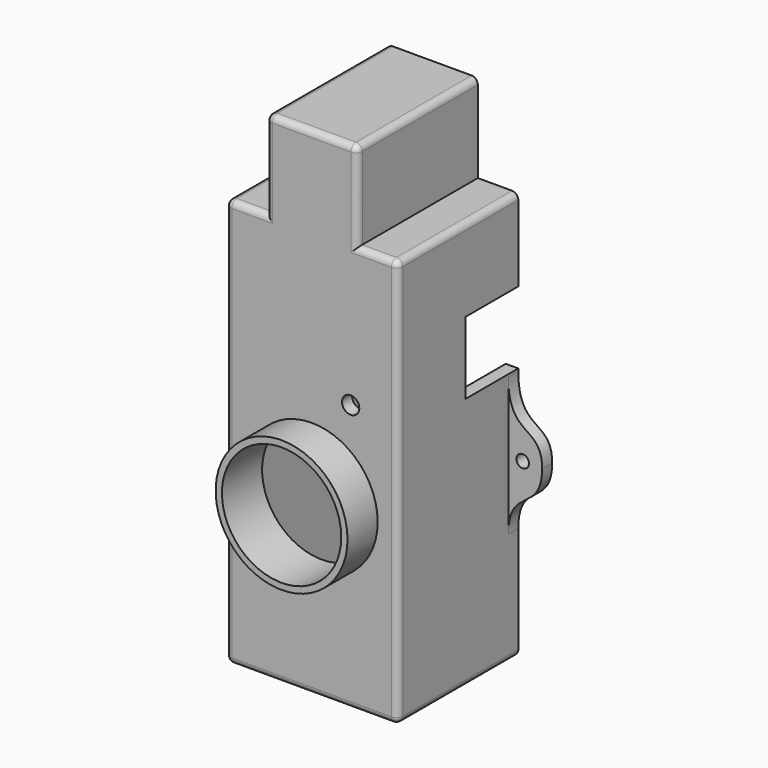
from build123d import *

# Parameters (mm, degrees)
F0_R        = 10.5
F0_R_2      = 1.375
F0_W        = 14.5
F0_H        = 14.06
F1_DEPTH    = 24
F2_T        = 2
F2_T3_DEPTH = 28
F0_R_3      = 9.5
F3_DEPTH    = 30
F0_R_4      = 1
F4_DEPTH    = 2
F5_R        = 1
F6_R        = 3.375
F7_DEPTH    = 22
F9_DEPTH    = 22
F10_W       = 10.5
F10_H       = 11.5
F11_DEPTH   = 2


# Not quite as in the source:
# - an extrude ends at something that could not be found from the text; its depth is read off the source's solid
# - a shell that OpenCascade refuses in one call is made with other operations: the cavity is built on its own and cut out


with BuildPart() as f1:
    # F0 (on Front) → F1 (new body)
    with BuildSketch(Plane.XZ):
        Polygon((-7.25, 32.5), (-13.7, 32.5), (-13.7, 7.4914984291), (-13.7, -14.5085015709), (-13.7, -32.5), (13.7, -32.5), (13.7, -14.5420665913), (13.7, 7.4579334087), (13.7, 32.5), (7.25, 32.5), align=None)
        with Locations((0, -4.91)):
            Circle(F0_R, mode=Mode.SUBTRACT)
        with Locations((6.2, 10.09)):
            Circle(F0_R_2, mode=Mode.SUBTRACT)
        with Locations((0, 39.53)):
            Rectangle(F0_W, F0_H)
    extrude(amount=F1_DEPTH)

    # F2: shell of thickness 2, made by hand


with BuildPart() as f2_core1:
    # F2_t2: copy of F1
    add(f1.part)

    # the walls: a layer under each face that stays
    f2_faces = [f2_core1.faces().sort_by_distance(p)[0] for p in [
        (-10.475, -12, 32.5),
        (-13.7, -12, 0),
        (0, -12, -32.5),
        (13.7, -12, 0),
        (10.475, -12, 32.5),
        (7.25, -12, 39.53),
        (0, -12, 46.56),
        (-7.25, -12, 39.53),
        (-10.5, -12, -4.91),
        (4.825, -12, 10.09),
        (0, -24, 7.03),
    ]]
    thicken(f2_faces, amount=-F2_T, mode=Mode.SUBTRACT)

    # F2_s4 → F2_t3 (cut)
    with BuildSketch(Plane.XZ.offset(-2)):
        Polygon((-7.27, 32.52), (-7.25, 30.5), (-5.25, 30.5), (-5.25, 32.5), align=None)
        Polygon((7.27, 32.52), (7.25, 30.5), (5.25, 30.5), (5.25, 32.5), align=None)
    extrude(amount=F2_T3_DEPTH, mode=Mode.SUBTRACT)


with BuildPart() as f1_1:
    add(f1.part)

    # what is left inside the walls is the cavity
    f2_cavity = [f2_core1.part.solids().sort_by_distance(p)[0] for p in [
        (0, -0.02, 14.513333),
        (0, -14.666667, -17.43),
    ]]
    add(f2_cavity, mode=Mode.SUBTRACT)

    # F0 (on Front) → F3 (join)
    with BuildSketch(Plane.XZ):
        with Locations((0, -4.91)):
            Circle(F0_R)
        with Locations((0, -4.91)):
            Circle(F0_R_3, mode=Mode.SUBTRACT)
    extrude(amount=F3_DEPTH)

    # F0 (on Front) → F4 (join)
    with BuildSketch(Plane.XZ):
        with BuildLine():
            Line((-13.7, -14.5085015709), (-13.7, 7.4914984291))
            add(Edge.make_bspline(
                [(-19.093351697, -3.5085015709), (-19.1026122295, 2.6293974578), (-13.7, -0.8116166133), (-13.7, 7.4914984291)],
                knots=[0, 0, 0, 0, 12.2510506704, 12.2510506704, 12.2510506704, 12.2510506704], degree=3))
            add(Edge.make_bspline(
                [(-19.093351697, -3.5085015709), (-19.0674920552, -9.0708802246), (-13.7, -6.7231292221), (-13.7, -14.5085015709)],
                knots=[0, 0, 0, 0, 12.2510506704, 12.2510506704, 12.2510506704, 12.2510506704], degree=3))
        make_face()
        with Locations((-16, -3.5420665913)):
            Circle(F0_R_4, mode=Mode.SUBTRACT)
        with BuildLine():
            add(Edge.make_bspline(
                [(19.0999998349, -3.5410547692), (19.0290823921, 2.4940823569), (13.7, -0.9160112299), (13.7, 7.4579334087)],
                knots=[0, 0, 0, 0, 12.2530706011, 12.2530706011, 12.2530706011, 12.2530706011], degree=3))
            Line((13.7, 7.4579334087), (13.7, -14.5420665913))
            add(Edge.make_bspline(
                [(19.0999998349, -3.5410547692), (19.0287452534, -10.2770104641), (13.7, -7.3807572052), (13.7, -14.5420665913)],
                knots=[0, 0, 0, 0, 12.2548871608, 12.2548871608, 12.2548871608, 12.2548871608], degree=3))
        make_face()
        with Locations((16, -3.5420665913)):
            Circle(F0_R_4, mode=Mode.SUBTRACT)
    extrude(amount=F4_DEPTH)

    # F5
    f5_edges = [f1_1.edges().sort_by_distance(p)[0] for p in [
        (13.7, -12, 32.5),
        (-13.7, -12, 32.5),
        (-13.7, -12, -32.5),
        (13.7, -12, -32.5),
        (7.25, -12, 46.56),
        (-7.25, -12, 46.56),
        (7.25, -24, 39.53),
        (-7.25, -24, 39.53),
        (-13.7, -24, 0),
        (13.7, -24, 0),
        (0, -24, -32.5),
        (-10.475, -24, 32.5),
        (10.475, -24, 32.5),
        (0, -24, 46.56),
    ]]
    fillet(f5_edges, radius=F5_R)

    # F6 (on face) → F7 (cut, through all)
    with BuildSketch(Plane(origin=(0, 0, 0), x_dir=(-1, 0, 0), z_dir=(0, 1, 0))):
        with Locations((-6.2, 10.09)):
            Circle(F6_R)
    extrude(amount=-F7_DEPTH, mode=Mode.SUBTRACT)

    # F8 (on face) → F9 (cut, through all)
    with BuildSketch(Plane(origin=(0, 0, 0), x_dir=(-1, 0, 0), z_dir=(0, 1, 0))):
        with BuildLine():
            ThreePointArc((-11.7, -9.31), (0, -17.41), (11.7, -9.31))
            Line((11.7, -9.31), (11.7, -0.51))
            ThreePointArc((11.7, -0.51), (0, 7.59), (-11.7, -0.51))
            Line((-11.7, -0.51), (-11.7, -9.31))
        make_face()
    extrude(amount=-F9_DEPTH, mode=Mode.SUBTRACT)

    # F10 (on face) → F11 (cut, through all)
    with BuildSketch(Plane.YZ.offset(13.7)):
        with Locations((-5.25, 13.6579334087)):
            Rectangle(F10_W, F10_H)
    extrude(amount=-F11_DEPTH, mode=Mode.SUBTRACT)


solid = f1_1.part
